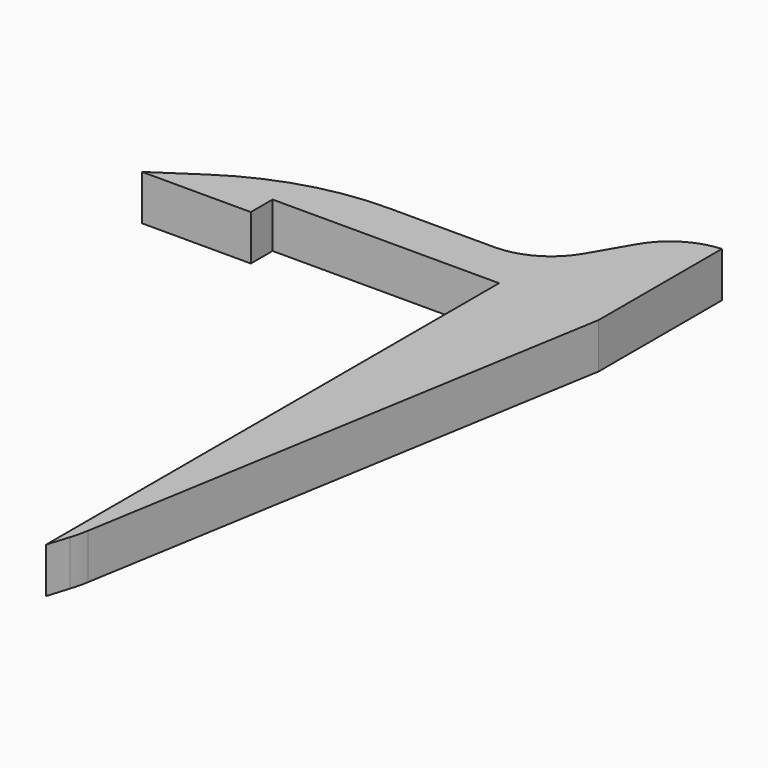
from build123d import *

# Parameters (mm, degrees)
F1_DEPTH    = 5
F2_T1_DEPTH = 5
F2_T3_DEPTH = 27.4743818089
F3_R        = 28.9973991458
F4_R        = 14.3918110757


# Not quite as in the source:
# - a fillet or chamfer that OpenCascade refuses, or shapes differently, is made with other operations: its cross-section is extruded or revolved along the edge and cut away or added


with BuildPart() as f1:
    # F0 (on Top) → F1 (new body)
    with BuildSketch(Plane.XY):
        Polygon((-25, 0), (0, 0), (0, -62.5), (1.0401320628, -59.1675673885), (11, 0), (11, 17), (7, 17), (0, 5), (-25, 5), (-37, -3), (-25, -3), align=None)
    extrude(amount=F1_DEPTH)

    # F2: fillet of radius 7.861186634 on 2 edges, made by hand

    # F2_s2 → F2_t1 (join)
    with BuildSketch(Plane.XY):
        with BuildLine():
            ThreePointArc((2.27509477, 8.9001624629), (-0.5998840547, 6.0444203344), (-4.5152323805, 5))
            Line((-4.5152323805, 5), (0, 5))
            Line((0, 5), (2.27509477, 8.9001624629))
        make_face()
    extrude(amount=F2_T1_DEPTH)

    # F2_s4 → F2_t3 (cut)
    with BuildSketch(Plane.XY.offset(-11.2371909045)):
        with BuildLine():
            ThreePointArc((11, 17), (7.3843664174, 15.838413937), (4.735162038, 13.1174206365))
            Line((4.735162038, 13.1174206365), (7, 17))
            Line((7, 17), (11, 17))
        make_face()
    extrude(amount=F2_T3_DEPTH, mode=Mode.SUBTRACT)

    # F3
    f3_edges = [f1.edges().sort_by_distance(p)[0] for p in [
        (-25, 5, 2.5),
    ]]
    fillet(f3_edges, radius=F3_R)

    # F4
    f4_edges = [f1.edges().sort_by_distance(p)[0] for p in [
        (1.040132, -59.167567, 2.5),
    ]]
    fillet(f4_edges, radius=F4_R)


solid = f1.part
